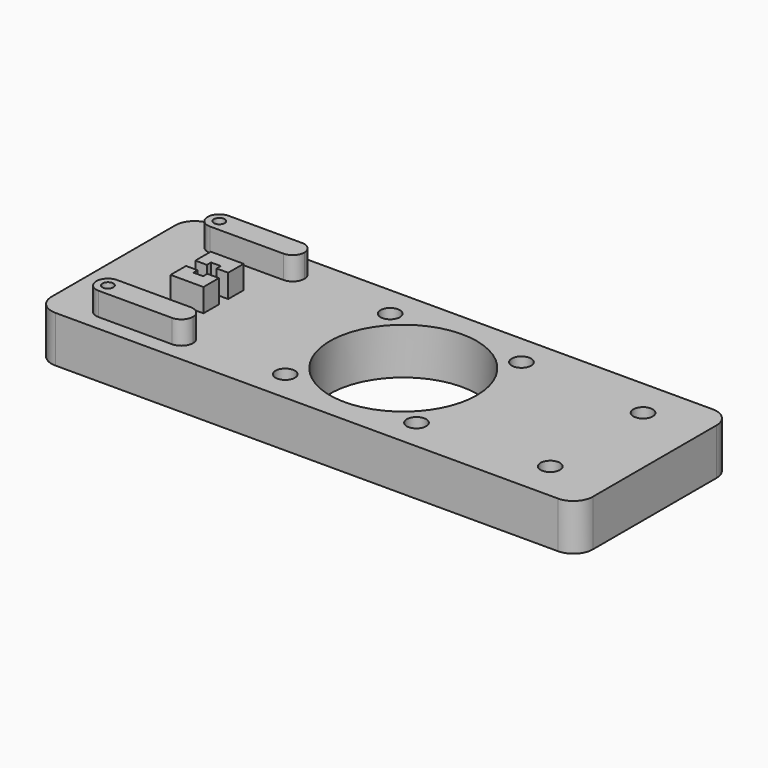
from build123d import *

# Parameters (mm, degrees)
F0_W     = 50
F0_H     = 50
F0_R     = 2.5
F0_R_2   = 19
F0_W_2   = 40
F1_DEPTH = 12
F2_R     = 5
F3_W     = 15
F3_H     = 6
F3_W_2   = 10
F4_DEPTH = 6
F5_R     = 2.99999
F6_R     = 1.4
F7_DEPTH = 18


# Not quite as in the source:
# - a fillet or chamfer is up to 0.001 mm smaller than in the source, because OpenCascade refuses the exact size


with BuildPart() as f1:
    # F0 (on Top) → F1 (new body)
    with BuildSketch(Plane.XY):
        Rectangle(F0_W, F0_H)
        with Locations((-16.9705627485, -16.9705627485)):
            Circle(F0_R, mode=Mode.SUBTRACT)
        with Locations((16.9705627485, -16.9705627485)):
            Circle(F0_R, mode=Mode.SUBTRACT)
        with Locations((-16.9705627485, 16.9705627485)):
            Circle(F0_R, mode=Mode.SUBTRACT)
        Circle(F0_R_2, mode=Mode.SUBTRACT)
        with Locations((16.9705627485, 16.9705627485)):
            Circle(F0_R, mode=Mode.SUBTRACT)
        with Locations((45, 0)):
            Rectangle(F0_W_2, F0_H)
        with Locations((50, -15)):
            Circle(F0_R, mode=Mode.SUBTRACT)
        with Locations((50, 15)):
            Circle(F0_R, mode=Mode.SUBTRACT)
        with Locations((-50, 0)):
            Rectangle(F0_W, F0_H)
    extrude(amount=F1_DEPTH)

    # F2
    f2_edges = [f1.edges().sort_by_distance(p)[0] for p in [
        (65, -25, 6),
        (65, 25, 6),
        (-75, -25, 6),
        (-75, 25, 6),
    ]]
    fillet(f2_edges, radius=F2_R)

    # F3 (on face) → F4 (join)
    with BuildSketch(Plane.XY.offset(12)):
        with Locations((-47.5, 18)):
            Rectangle(F3_W, F3_H)
        with Locations((-60, 18)):
            Rectangle(F3_W_2, F3_H)
        with Locations((-47.5, -18)):
            Rectangle(F3_W, F3_H)
        with Locations((-60, -18)):
            Rectangle(F3_W_2, F3_H)
        Polygon((-46.5, 6.5), (-55, 6.5), (-55, 1.5), (-52, 1.5), (-52, 2.85), (-49.5, 2.85), (-49.5, 1.5), (-46.5, 1.5), align=None)
        Polygon((-46.5, -6.5), (-46.5, -1.5), (-49.5, -1.5), (-49.5, -2.85), (-52, -2.85), (-52, -1.5), (-55, -1.5), (-55, -6.5), align=None)
    extrude(amount=F4_DEPTH)

    # F5 (radius 3 in the source; OpenCascade refuses exactly that, so slightly less here)
    f5_edges = [f1.edges().sort_by_distance(p)[0] for p in [
        (-65, 21, 15),
        (-65, 15, 15),
        (-40, 15, 15),
        (-65, -15, 15),
        (-65, -21, 15),
        (-40, -21, 15),
        (-40, -15, 15),
        (-40, 21, 15),
    ]]
    fillet(f5_edges, radius=F5_R)

    # F6 (on face) → F7 (cut, through all)
    with BuildSketch(Plane.XY.offset(18)):
        with Locations((-62, 18)):
            Circle(F6_R)
        with Locations((-62, -18)):
            Circle(F6_R)
    extrude(amount=-F7_DEPTH, mode=Mode.SUBTRACT)


solid = f1.part
